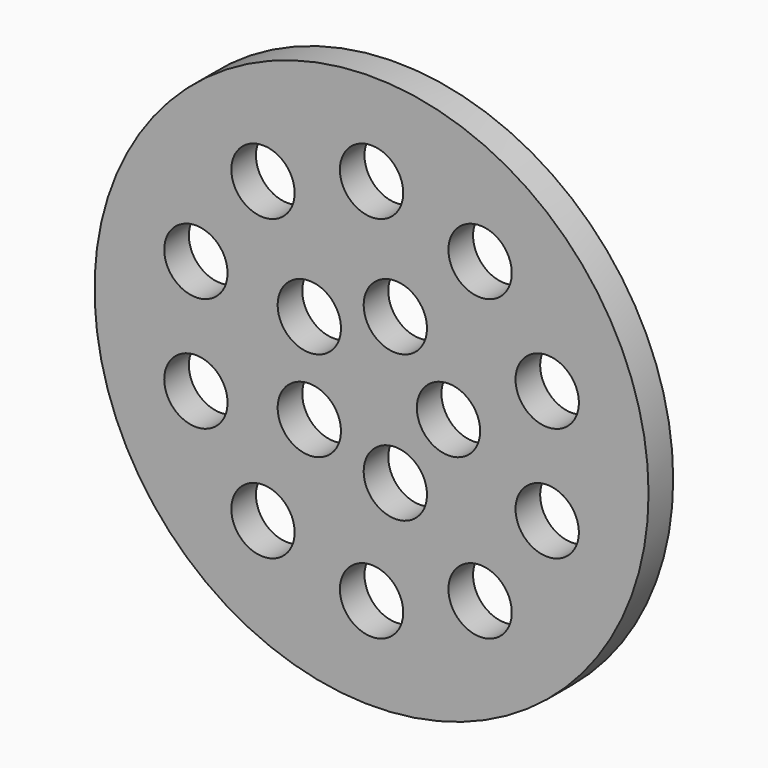
from build123d import *

# Parameters (mm, degrees)
F0_R     = 9
F1_DEPTH = 1
F3_D     = 2.0574
F3_DEPTH = 15
F3_TIP   = 0.6181053188


# Not quite as in the source:
# - a feature names something its author has since deleted; it is built from what else it names


with BuildPart() as f1:
    # F0 (on Front) → F1 (new body)
    with BuildSketch(Plane.XZ):
        Circle(F0_R)
    extrude(amount=F1_DEPTH)

    # F3
    with Locations(Plane.XZ.offset(1)):
        with Locations((-3.5267115138, 4.8541019662), (-5.7063390978, 1.8541019662), (-5.7063390978, -1.8541019662), (-3.5267115138, -4.8541019662), (0, -6), (3.5267115138, -4.8541019662), (5.7063390978, -1.8541019662), (0, 6), (-2.0225424859, 1.4694631307), (-2.0225424859, -1.4694631307), (0.7725424859, -2.3776412907), (2.5, 0), (0.7725424859, 2.3776412907), (3.5267115138, 4.8541019662), (5.7063390978, 1.8541019662)):
            Hole(F3_D / 2, depth=F3_DEPTH)
            with Locations((0, 0, -(F3_DEPTH + F3_TIP / 2))):  # 118° drill point
                Cone(0, F3_D / 2, F3_TIP, mode=Mode.SUBTRACT)


solid = f1.part
